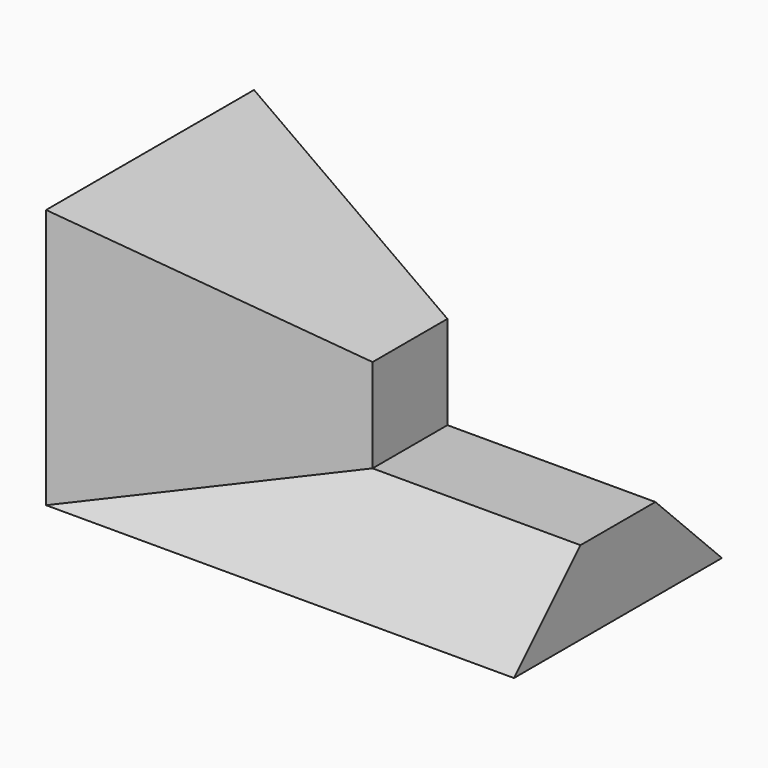
from build123d import *

# Parameters (mm, degrees)
F0_W     = 63.5
F0_H     = 63.5
F1_DEPTH = 31.75
F2_SIZE2 = 63.49999
F2_SIZE  = 20.31999
F4_DEPTH = 114.3


# Not quite as in the source:
# - a fillet or chamfer is up to 0.001 mm smaller than in the source, because OpenCascade refuses the exact size


with BuildPart() as f1:
    # F0 (on Right) → F1 (new body, symmetric)
    with BuildSketch(Plane.YZ):
        Rectangle(F0_W, F0_H)
    extrude(amount=F1_DEPTH, both=True)

    # F2 (size 20.32 and 63.5 in the source; OpenCascade refuses exactly that, so slightly less here)
    f2_edges = [f1.edges().sort_by_distance(p)[0] for p in [
        (31.75, -31.75, 0),
        (31.75, 0, 31.75),
        (31.75, 31.75, 0),
        (31.75, 0, -31.75),
    ]]
    f2_side = f1.faces().sort_by_distance((31.75, 0, 0))[0]
    chamfer(f2_edges, length=F2_SIZE, length2=F2_SIZE2, reference=f2_side)

    # F3 (on face) → F4 (join)
    with BuildSketch(Plane(origin=(-31.75, 0, 0), x_dir=(0, -1, 0), z_dir=(-1, 0, 0))):
        Polygon((-31.75, -31.75), (31.75, -31.75), (11.43, -11.43), (-11.43, -11.43), align=None)
    extrude(amount=-F4_DEPTH)


solid = f1.part
